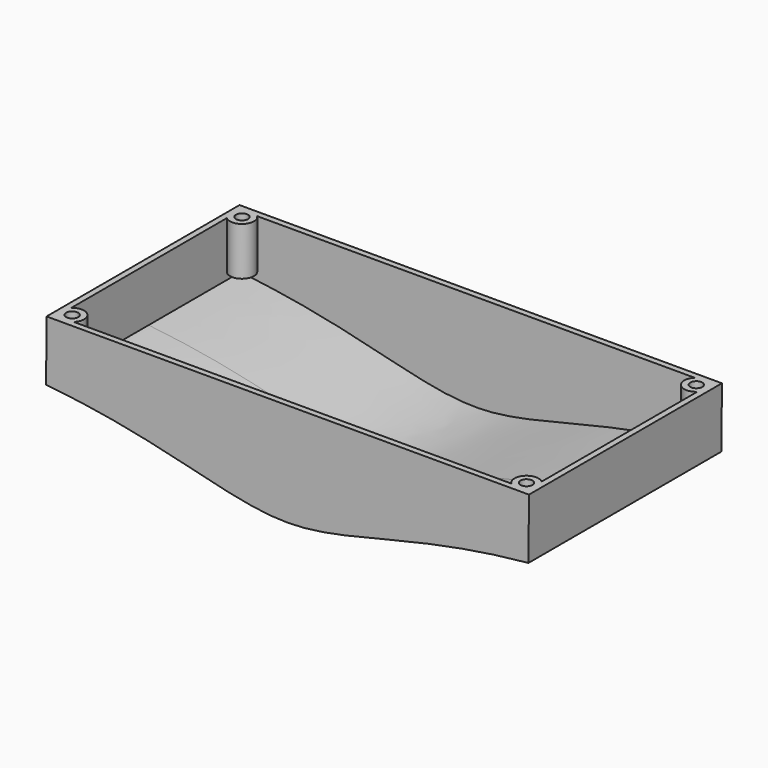
from build123d import *

# Parameters (mm, degrees)
F1_DEPTH = 50
F2_T     = -2.5
F3_R     = 4.9550081524
F3_R_2   = 2.5
F4_DEPTH = 20


with BuildPart() as f1:
    # F0 (on Front) → F1 (new body, symmetric)
    with BuildSketch(Plane.XZ):
        with BuildLine():
            Line((100, 20), (-100, 20))
            Line((-100, 20), (-100.1966984122, -5))
            add(Edge.make_bspline(
                [(-100.1966984122, -5), (-50, -10.014916776), (-0.095335689, -35.6705608011), (50, -9.7627513964), (99.8033015878, -5)],
                knots=[0, 0, 0, 0, 0.500476678, 1, 1, 1, 1], degree=3))
            Line((99.8033015878, -5), (100, 20))
        make_face()
    extrude(amount=F1_DEPTH, both=True)

    # F2
    f2_openings = [f1.faces().sort_by_distance(p)[0] for p in [
        (0, 0, 20),
    ]]
    offset(amount=F2_T, openings=f2_openings, kind=Kind.INTERSECTION)



with BuildPart() as f4:
    # F3 (on Top) → F4 (new body)
    with BuildSketch(Plane.XY):
        with Locations((-94.1810160875, -44.0020188689)):
            Circle(F3_R)
        with Locations((-94.1810160875, -44.0020188689)):
            Circle(F3_R_2, mode=Mode.SUBTRACT)
    extrude(amount=F4_DEPTH)


with BuildPart() as f5_1:
    # F5: instance of F4
    add(f4.part.mirror(Plane.YZ))


with BuildPart() as f1_1:
    add(f1.part)

    add(f4.part)  # F6 merges F4

    add(f5_1.part)  # F6 merges F5_1
    # F6: F4, F5_1 across plane
    add(f4.part.mirror(Plane.XZ))
    add(f5_1.part.mirror(Plane.XZ))


solid = f1_1.part
